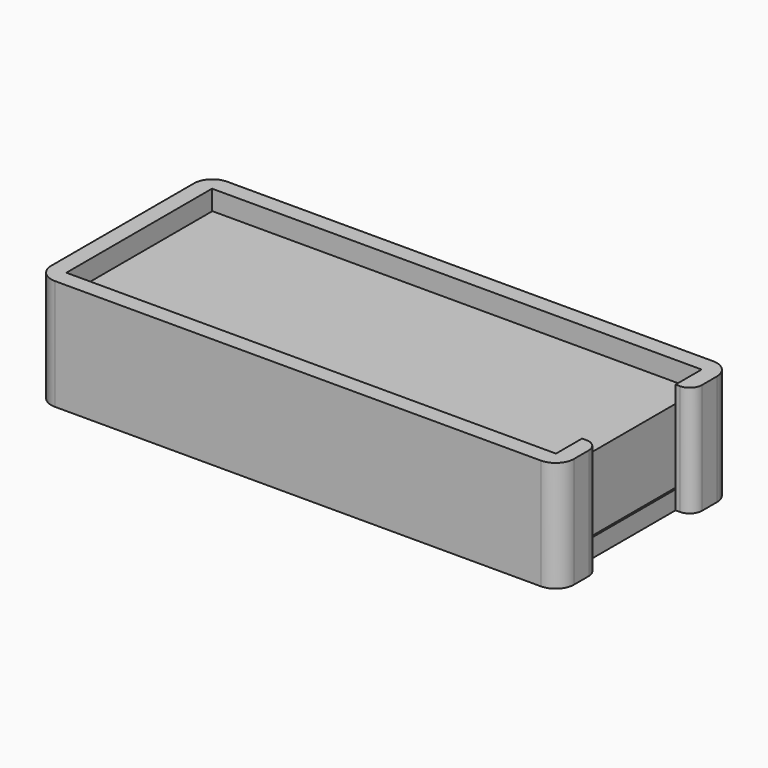
from build123d import *

# Parameters (mm, degrees)
F0_W     = 79
F0_H     = 29
F1_DEPTH = 12
F2_W     = 85
F2_H     = 35
F2_W_2   = 79.6
F2_H_2   = 29.6
F3_DEPTH = 15
F4_W     = 85
F4_H     = 35
F5_DEPTH = 3
F6_W     = 2.7
F6_H     = 19
F7_DEPTH = 25
F8_R     = 2
F9_R     = 3


with BuildPart() as f1:
    # F0 (on Top) → F1 (new body)
    with BuildSketch(Plane.XY):
        Rectangle(F0_W, F0_H)
    extrude(amount=F1_DEPTH)


with BuildPart() as f3:
    # F2 (on Top) → F3 (new body)
    with BuildSketch(Plane.XY):
        Rectangle(F2_W, F2_H)
        Rectangle(F2_W_2, F2_H_2, mode=Mode.SUBTRACT)
    extrude(amount=F3_DEPTH)

    # F4 (on face) → F5 (join)
    with BuildSketch(Plane(origin=(0, 0, 0), x_dir=(1, 0, 0), z_dir=(0, 0, -1))):
        Rectangle(F4_W, F4_H)
    extrude(amount=F5_DEPTH)

    # F6 (on face) → F7 (cut)
    with BuildSketch(Plane.XY.offset(15)):
        with Locations((41.15, 0)):
            Rectangle(F6_W, F6_H)
    extrude(amount=-F7_DEPTH, mode=Mode.SUBTRACT)

    # F8
    f8_edges = [f3.edges().sort_by_distance(p)[0] for p in [
        (42.5, -9.5, 6),
        (42.5, 9.5, 6),
    ]]
    fillet(f8_edges, radius=F8_R)

    # F9
    f9_edges = [f3.edges().sort_by_distance(p)[0] for p in [
        (42.5, -17.5, 6),
        (-42.5, -17.5, 6),
        (-42.5, 17.5, 6),
        (42.5, 17.5, 6),
    ]]
    fillet(f9_edges, radius=F9_R)


solid = Compound([f1.part, f3.part])
